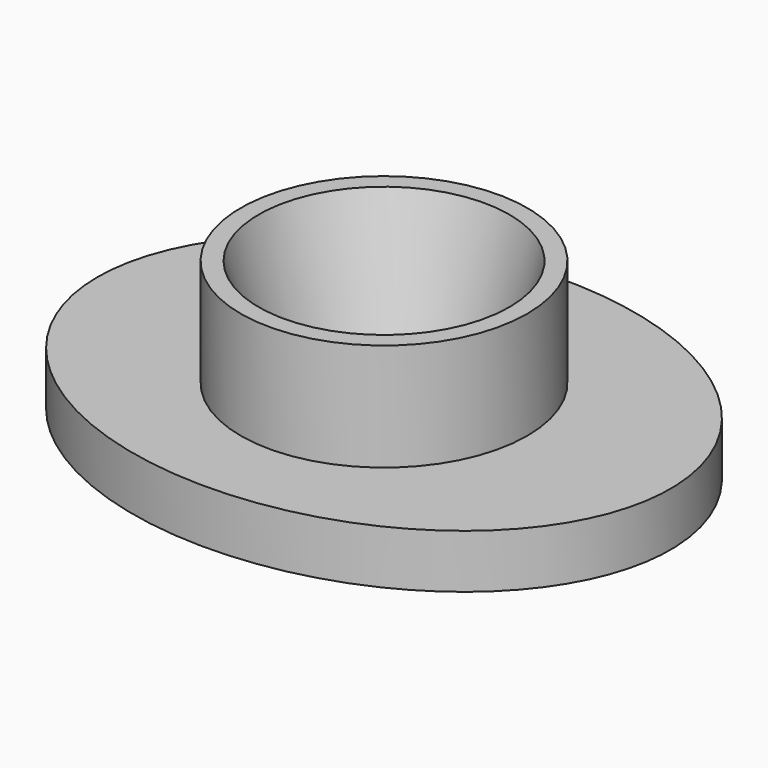
from build123d import *

# Parameters (mm, degrees)
F0_R     = 8
F1_DEPTH = 3
F0_R_2   = 7
F2_DEPTH = 9
F0_R_3   = 4.5
F3_DEPTH = 9
F4_DEPTH = 25
F5_SIZE2 = 2.49999
F5_SIZE  = 8.99999


# Not quite as in the source:
# - a fillet or chamfer is up to 0.001 mm smaller than in the source, because OpenCascade refuses the exact size


with BuildPart() as f1:
    # F0 (on Top) → F1 (new body)
    with BuildSketch(Plane.XY):
        with BuildLine():
            add(Edge.make_bspline(
                [(-16, 0), (-16, -21.6506350946), (8, -10.8253175473), (32, 0), (8, 10.8253175473), (-16, 21.6506350946), (-16, 0)],
                knots=[0, 0, 0, 2.0943951024, 2.0943951024, 4.1887902048, 4.1887902048, 6.2831853072, 6.2831853072, 6.2831853072], degree=2, weights=[1, 0.5, 1, 0.5, 1, 0.5, 1]))
        make_face()
        Circle(F0_R, mode=Mode.SUBTRACT)
    extrude(amount=F1_DEPTH)

    # F0 (on Top) → F2 (join)
    with BuildSketch(Plane.XY):
        Circle(F0_R)
        Circle(F0_R_2, mode=Mode.SUBTRACT)
    extrude(amount=F2_DEPTH)

    # F0 (on Top) → F4 (cut)
    with BuildSketch(Plane.XY):
        Circle(F0_R_3)
    extrude(amount=-F4_DEPTH, mode=Mode.SUBTRACT)


with BuildPart() as f3:
    # F0 (on Top) → F3 (new body, through all)
    with BuildSketch(Plane.XY):
        Circle(F0_R_2)
        Circle(F0_R_3, mode=Mode.SUBTRACT)
    extrude(amount=F3_DEPTH)

    # F5 (size 9 and 2.5 in the source; OpenCascade refuses exactly that, so slightly less here)
    f5_edges = [f3.edges().sort_by_distance(p)[0] for p in [
        (-4.5, 0, 9),
    ]]
    f5_side = f3.faces().sort_by_distance((-4.5, 0, 4.5))[0]
    chamfer(f5_edges, length=F5_SIZE, length2=F5_SIZE2, reference=f5_side)


solid = Compound([f1.part, f3.part])
